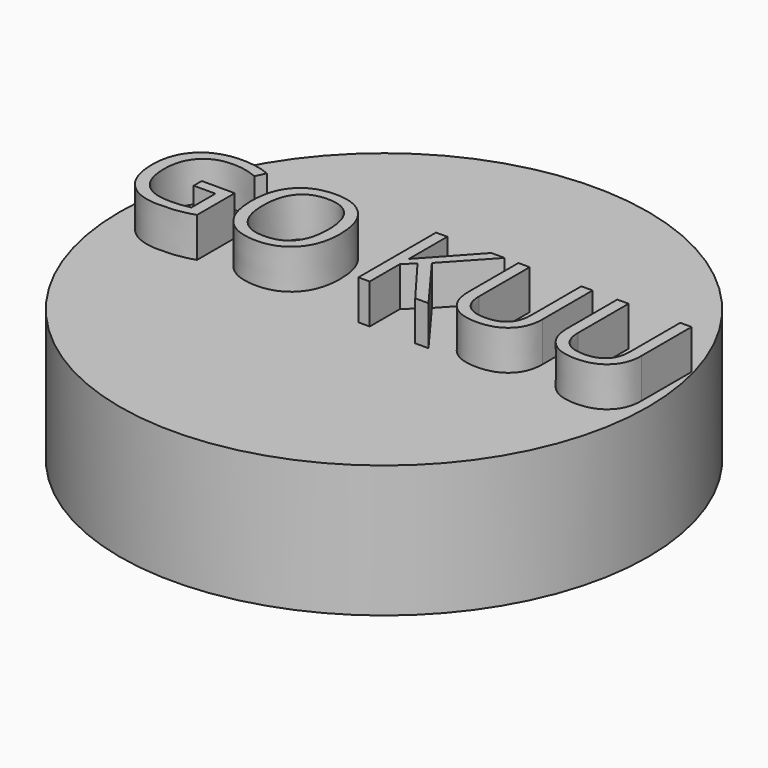
from build123d import *

# Parameters (mm, degrees)
F0_R         = 25.4
F1_DEPTH     = 12.7
F2_TEXT_SIZE = 13.064252423
F3_DEPTH     = 3.81


# Not quite as in the source:
# - Text() gives the source's letters only with a copy of the font that has no kerning and outlines rounded to 1/6400 em; it was checked with that copy


with BuildPart() as f1:
    # F0 (on Top) → F1 (new body)
    with BuildSketch(Plane.XY):
        Circle(F0_R)
    extrude(amount=F1_DEPTH)

    # F2 (on face) → F3 (join)
    with BuildSketch(Plane.XY.offset(12.7)):
        with Locations((-24.5392967097, -2.8501259166)):
            Text('GO KUU', F2_TEXT_SIZE, font='Open Sans', text_align=(TextAlign.LEFT, TextAlign.BOTTOM))
    extrude(amount=F3_DEPTH)


solid = f1.part
